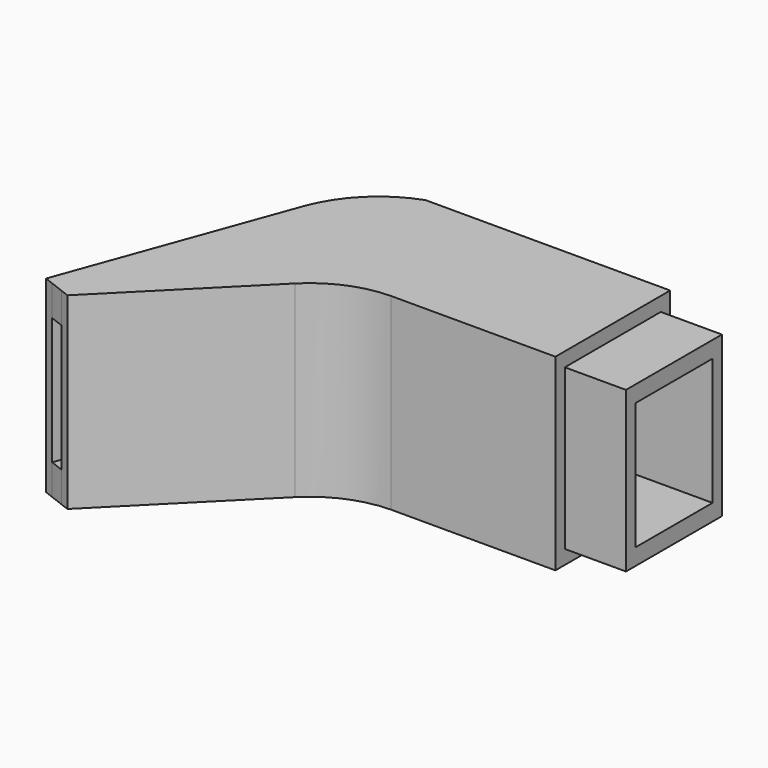
from build123d import *

# Parameters (mm, degrees)
F0_W     = 17.5
F0_H     = 1.25
F1_DEPTH = 10
F0_H_2   = 10.25
F2_DEPTH = 10
F0_W_2   = 6.5
F3_DEPTH = 8.5
F4_DEPTH = 6.75
F5_DEPTH = 6.75


# Not quite as in the source:
# - a feature names something its author has since deleted; it is built from what else it names


with BuildPart() as f1:
    # F0 (on Top) → F1 (new body, symmetric)
    with BuildSketch(Plane.XY):
        with Locations((20.0137786908, 13.375)):
            Rectangle(F0_W, F0_H)
        with Locations((20.0137786908, 12.125)):
            Rectangle(F0_W, F0_H)
        with BuildLine():
            Line((2.7637786908, 11.5), (11.2637786908, 11.5))
            Line((11.2637786908, 11.5), (11.2637786908, 12.75))
            Line((11.2637786908, 12.75), (11.2637786908, 14))
            Line((11.2637786908, 14), (2.7637786908, 14))
            ThreePointArc((2.7637786908, 14), (-1.6624935941, 11.2110263052), (-4.4814392939, 6.8037816159))
            Line((-4.4814392939, 6.8037816159), (-13.0372270502, -16.686609949))
            Line((-13.0372270502, -16.686609949), (-12.1037272591, -17.0451878901))
            Line((-12.1037272591, -17.0451878901), (-3.7917014922, 5.0309925083))
            ThreePointArc((-3.7917014922, 5.0309925083), (-1.2235822128, 8.9846027287), (2.7637786908, 11.5))
        make_face()
    extrude(amount=F1_DEPTH, both=True)



with BuildPart() as f1b:
    # F0 (on Top) → F1, piece 2 (new body, symmetric)
    with BuildSketch(Plane.XY):
        with Locations((20.0137786908, 0.625)):
            Rectangle(F0_W, F0_H)
        with Locations((20.0137786908, -0.625)):
            Rectangle(F0_W, F0_H)
        with BuildLine():
            Line((11.2637786908, -1.25), (11.2637786908, 0))
            Line((11.2637786908, 0), (11.2637786908, 1.25))
            ThreePointArc((11.2637786908, 1.25), (6.1499097664, -0.1712613654), (1.9326170674, -3.3940057761))
            Line((1.9326170674, -3.3940057761), (-10.7034775723, -17.5830548019))
            Line((-10.7034775723, -17.5830548019), (-9.7699777812, -17.9416327431))
            Line((-9.7699777812, -17.9416327431), (3.6421700758, -4.483761817))
            ThreePointArc((3.6421700758, -4.483761817), (7.1371242658, -2.1224581239), (11.2637786908, -1.25))
        make_face()
    extrude(amount=F1_DEPTH, both=True)


with BuildPart() as f1_1:
    add(f1.part)

    add(f1b.part)  # F2 merges F1b
    # F0 (on Top) → F2 (join, symmetric)
    with BuildSketch(Plane.XY):
        with Locations((20.0137786908, 6.375)):
            Rectangle(F0_W, F0_H_2)
        with BuildLine():
            ThreePointArc((1.9326170674, -3.3940057761), (6.1499097664, -0.1712613654), (11.2637786908, 1.25))
            Line((11.2637786908, 1.25), (11.2637786908, 11.5))
            Line((11.2637786908, 11.5), (2.7637786908, 11.5))
            ThreePointArc((2.7637786908, 11.5), (-1.2235822128, 8.9846027287), (-3.7917014922, 5.0309925083))
            Line((-3.7917014922, 5.0309925083), (-12.1037272591, -17.0451878901))
            Line((-12.1037272591, -17.0451878901), (-10.7034775723, -17.5830548019))
            Line((-10.7034775723, -17.5830548019), (1.9326170674, -3.3940057761))
        make_face()
    extrude(amount=F2_DEPTH, both=True)

    # F0 (on Top) → F3 (join, symmetric)
    with BuildSketch(Plane.XY):
        with Locations((32.0137786908, 12.125)):
            Rectangle(F0_W_2, F0_H)
        with Locations((32.0137786908, 6.375)):
            Rectangle(F0_W_2, F0_H_2)
        with Locations((32.0137786908, 0.625)):
            Rectangle(F0_W_2, F0_H)
    extrude(amount=F3_DEPTH, both=True)

    # F0 (on Top) → F4 (cut, symmetric)
    with BuildSketch(Plane.XY):
        with Locations((20.0137786908, 6.375)):
            Rectangle(F0_W, F0_H_2)
        with BuildLine():
            ThreePointArc((1.9326170674, -3.3940057761), (6.1499097664, -0.1712613654), (11.2637786908, 1.25))
            Line((11.2637786908, 1.25), (11.2637786908, 11.5))
            Line((11.2637786908, 11.5), (2.7637786908, 11.5))
            ThreePointArc((2.7637786908, 11.5), (-1.2235822128, 8.9846027287), (-3.7917014922, 5.0309925083))
            Line((-3.7917014922, 5.0309925083), (-12.1037272591, -17.0451878901))
            Line((-12.1037272591, -17.0451878901), (-10.7034775723, -17.5830548019))
            Line((-10.7034775723, -17.5830548019), (1.9326170674, -3.3940057761))
        make_face()
    extrude(amount=F4_DEPTH, both=True, mode=Mode.SUBTRACT)

    # F0 (on Top) → F5 (cut, symmetric)
    with BuildSketch(Plane.XY):
        with Locations((32.0137786908, 6.375)):
            Rectangle(F0_W_2, F0_H_2)
    extrude(amount=F5_DEPTH, both=True, mode=Mode.SUBTRACT)


solid = f1_1.part
